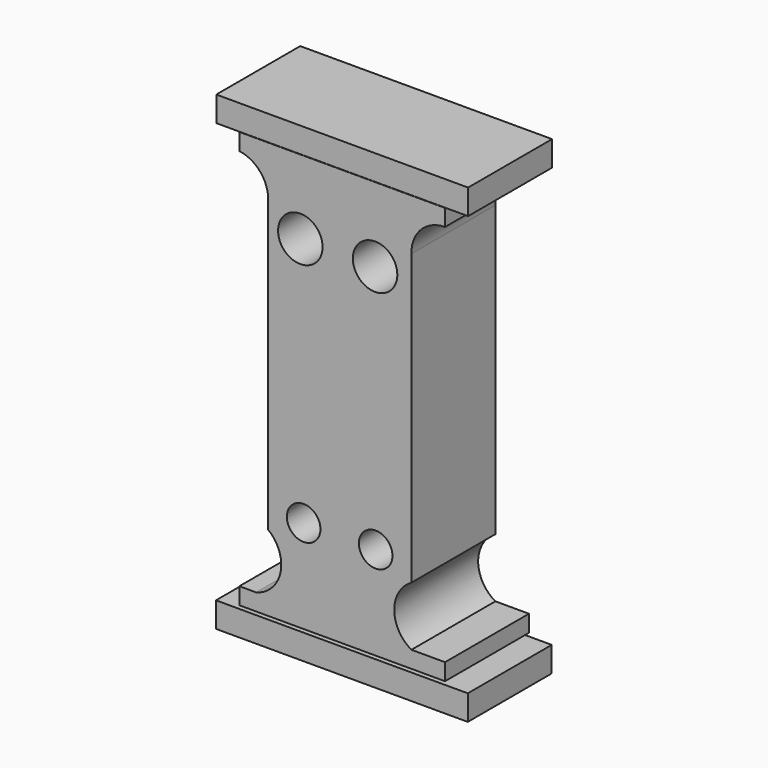
from build123d import *

# Parameters (mm, degrees)
F0_W     = 60
F0_H     = 6
F1_DEPTH = 25
F0_W_2   = 49
F0_H_2   = 4
F0_R     = 4
F0_R_2   = 5.3


with BuildPart() as f1:
    # F0 (on Front) → F1 (new body)
    with BuildSketch(Plane.XZ):
        with Locations((-0.0771296024, -54.9107142985)):
            Rectangle(F0_W, F0_H)
    extrude(amount=F1_DEPTH)


with BuildPart() as f1b:
    # F0 (on Front) → F1, piece 2 (new body)
    with BuildSketch(Plane.XZ):
        with Locations((0, 51.1985905468)):
            Rectangle(F0_W, F0_H)
    extrude(amount=F1_DEPTH)


with BuildPart() as f1c:
    # F0 (on Front) → F1, piece 3 (new body)
    with BuildSketch(Plane.XZ):
        with Locations((0, 46.1378805339)):
            Rectangle(F0_W_2, F0_H_2)
        with BuildLine():
            ThreePointArc((24.5, -47.1425395012), (20.4991438354, -48.1999383489), (16.4982876707, -47.1425395012))
            Line((16.4982876707, -47.1425395012), (-20.5270550462, -47.1425395012))
            ThreePointArc((-20.5270550462, -47.1425395012), (-22.5135275231, -47.3930926113), (-24.5, -47.1425395012))
            Line((-24.5, -47.1425395012), (-24.5, -51.1425395012))
            Line((-24.5, -51.1425395012), (24.5, -51.1425395012))
            Line((24.5, -51.1425395012), (24.5, -47.1425395012))
        make_face()
        with BuildLine():
            ThreePointArc((16.4982876707, 35.9380108601), (18.7701769789, 41.7251304893), (24.5, 44.1378805339))
            Line((24.5, 44.1378805339), (-24.5, 44.1378805339))
            ThreePointArc((-24.5, 44.1378805339), (-19.4885163945, 41.3571658308), (-17.6230133544, 35.9380108601))
            Line((-17.6230133544, 35.9380108601), (16.4982876707, 35.9380108601))
        make_face()
        with BuildLine():
            ThreePointArc((-24.5, -47.1425395012), (-22.5135275231, -47.3930926113), (-20.5270550462, -47.1425395012))
            Line((-20.5270550462, -47.1425395012), (-24.5, -47.1425395012))
        make_face()
        with BuildLine():
            Line((24.5, -47.1425395012), (16.4982876707, -47.1425395012))
            ThreePointArc((16.4982876707, -47.1425395012), (20.4991438354, -48.1999383489), (24.5, -47.1425395012))
        make_face()
        with BuildLine():
            Line((16.4982876707, -33.0619891399), (16.4982876707, 35.9380108601))
            Line((16.4982876707, 35.9380108601), (-17.6230133544, 35.9380108601))
            Line((-17.6230133544, 35.9380108601), (-17.6230133544, -33.0619891399))
            ThreePointArc((-17.6230133544, -33.0619891399), (-14.678432696, -41.0090409552), (-20.5270550462, -47.1425395012))
            Line((-20.5270550462, -47.1425395012), (16.4982876707, -47.1425395012))
            ThreePointArc((16.4982876707, -47.1425395012), (12.401469807, -40.1022643205), (16.4982876707, -33.0619891399))
        make_face()
        with Locations((-9.1818850487, -28.8949348032)):
            Circle(F0_R, mode=Mode.SUBTRACT)
        with Locations((7.9746739939, -28.8949348032)):
            Circle(F0_R, mode=Mode.SUBTRACT)
        with Locations((-9.9784871563, 30.4424017668)):
            Circle(F0_R_2, mode=Mode.SUBTRACT)
        with Locations((7.8374212608, 30.3981341422)):
            Circle(F0_R_2, mode=Mode.SUBTRACT)
    extrude(amount=F1_DEPTH)


solid = Compound([f1.part, f1b.part, f1c.part])
